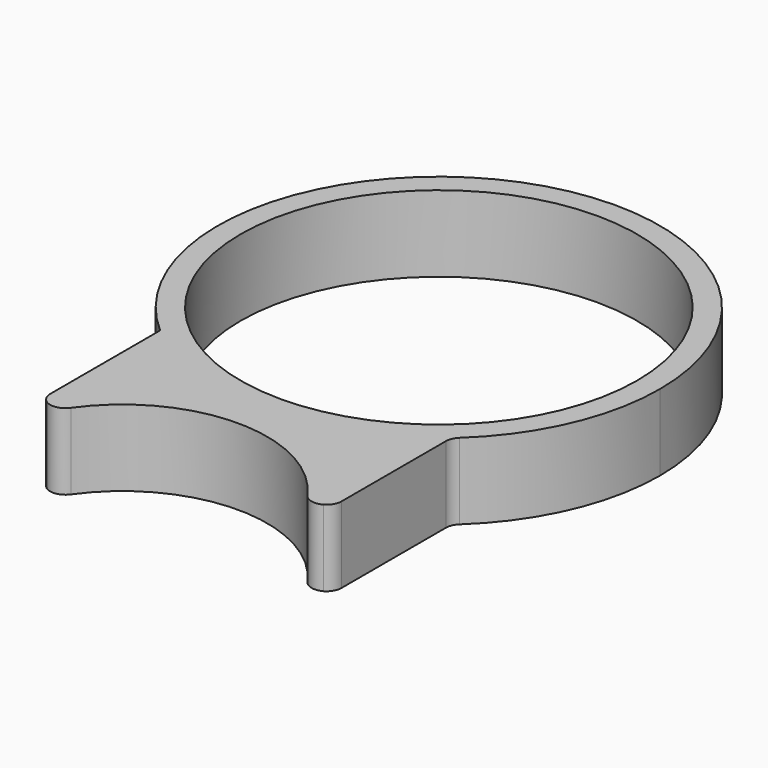
from build123d import *

# Parameters (mm, degrees)
F0_R        = 26
F1_DEPTH    = 10
F2_T1_DEPTH = 10
F2_T3_DEPTH = 15.7735026919
F2_T5_DEPTH = 19.5643999635


# Not quite as in the source:
# - a fillet or chamfer that OpenCascade refuses, or shapes differently, is made with other operations: its cross-section is extruded or revolved along the edge and cut away or added


with BuildPart() as f1:
    # F0 (on Top) → F1 (new body)
    with BuildSketch(Plane.XY):
        with BuildLine():
            ThreePointArc((19.0958601534, -21.8254009127), (26.4081421578, -11.9837401413), (29, 0))
            ThreePointArc((29, 0), (-11.9837401413, 26.4081421578), (-19.0958601534, -21.8254009127))
            ThreePointArc((-19.0958601534, -21.8254009127), (0, -29), (19.0958601534, -21.8254009127))
        make_face()
        Circle(F0_R, mode=Mode.SUBTRACT)
        with BuildLine():
            ThreePointArc((19.0958601534, -21.8254009127), (0, -29), (-19.0958601534, -21.8254009127))
            Line((-19.0958601534, -21.8254009127), (-19.0958601534, -40.975))
            ThreePointArc((-19.0958601534, -40.975), (0, -29.8996567452), (19.0958601534, -40.975))
            Line((19.0958601534, -40.975), (19.0958601534, -21.8254009127))
        make_face()
        with BuildLine():
            ThreePointArc((19.0958601534, -40.975), (0, -29.8996567452), (-19.0958601534, -40.975))
            Line((-19.0958601534, -40.975), (-16.4977839421, -42.475))
            ThreePointArc((-16.4977839421, -42.475), (0, -32.8996021136), (16.4977839421, -42.475))
            Line((16.4977839421, -42.475), (19.0958601534, -40.975))
        make_face()
    extrude(amount=F1_DEPTH)

    # F2: fillet of radius 2 on 5 edges, made by hand

    # F2_s2 → F2_t1 (join)
    with BuildSketch(Plane.XY):
        with BuildLine():
            ThreePointArc((19.7348369177, -21.2493814458), (19.2625507863, -21.9154958064), (19.0958601534, -22.7148560283))
            Line((19.0958601534, -22.7148560283), (19.0958601534, -21.8254009127))
            ThreePointArc((19.0958601534, -21.8254009127), (19.4174846045, -21.5397607144), (19.7348369177, -21.2493814458))
        make_face()
    extrude(amount=F2_T1_DEPTH)

    # F2_s4 → F2_t3 (cut)
    with BuildSketch(Plane.XY.offset(-2.8867513459)):
        with BuildLine():
            ThreePointArc((-19.0958601534, -39.8202994616), (-18.827910961, -40.8202994616), (-18.0958601534, -41.5523502692))
            Line((-18.0958601534, -41.5523502692), (-19.0958601534, -40.975))
            Line((-19.0958601534, -40.975), (-19.0958601534, -39.8202994616))
        make_face()
        with BuildLine():
            ThreePointArc((18.0958601534, -41.5523502692), (18.827910961, -40.8202994616), (19.0958601534, -39.8202994616))
            Line((19.0958601534, -39.8202994616), (19.0958601534, -40.975))
            Line((19.0958601534, -40.975), (18.0958601534, -41.5523502692))
        make_face()
    extrude(amount=F2_T3_DEPTH, mode=Mode.SUBTRACT)

    # F2_s6 → F2_t5 (cut)
    with BuildSketch(Plane.XY.offset(-4.7821999818)):
        with BuildLine():
            ThreePointArc((-18.1543866102, -41.5185600036), (-16.7253721793, -41.7399540041), (-15.5206355044, -40.940137093))
            ThreePointArc((-15.5206355044, -40.940137093), (-16.0275933003, -41.6958649061), (-16.4977839421, -42.475))
            Line((-16.4977839421, -42.475), (-18.1543866102, -41.5185600036))
        make_face()
        with BuildLine():
            ThreePointArc((15.5206355044, -40.940137093), (16.7253721793, -41.7399540041), (18.1543866102, -41.5185600036))
            Line((18.1543866102, -41.5185600036), (16.4977839421, -42.475))
            ThreePointArc((16.4977839421, -42.475), (16.0275933003, -41.6958649061), (15.5206355044, -40.940137093))
        make_face()
    extrude(amount=F2_T5_DEPTH, mode=Mode.SUBTRACT)


solid = f1.part
